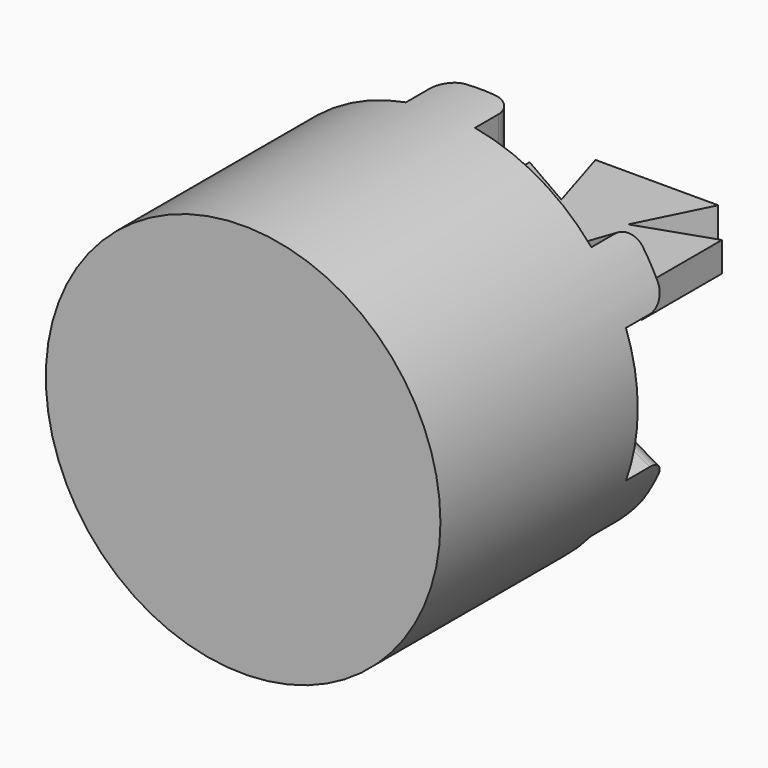
from build123d import *

# Parameters (mm, degrees)
F0_R     = 20
F1_DEPTH = 30
F2_R     = 15
F3_DEPTH = 10
F5_DEPTH = 5
F6_R     = 2
F8_DEPTH = 3


# Not quite as in the source:
# - a feature names something its author has since deleted; it is built from what else it names


with BuildPart() as f1:
    # F0 (on Front) → F1 (new body)
    with BuildSketch(Plane.XZ):
        Circle(F0_R)
    extrude(amount=-F1_DEPTH)

    # F2 (on face) → F3 (cut)
    with BuildSketch(Plane(origin=(0, 30, 0), x_dir=(-1, 0, 0), z_dir=(0, 1, 0))):
        Circle(F2_R)
    extrude(amount=-F3_DEPTH, mode=Mode.SUBTRACT)

    # F4 (on face) → F5 (cut)
    with BuildSketch(Plane(origin=(0, 30, 0), x_dir=(-1, 0, 0), z_dir=(0, 1, 0))):
        with BuildLine():
            Line((-3.5, -19.6913686675), (-3.5, -14.5859521458))
            ThreePointArc((-3.5, -14.5859521458), (-7.5, -12.9903810568), (-10.8818050967, -10.3240649862))
            Line((-10.8818050967, -10.3240649862), (-15.3032255014, -12.876773247))
            ThreePointArc((-15.3032255014, -12.876773247), (-10, -17.3205080757), (-3.5, -19.6913686675))
        make_face()
        with BuildLine():
            Line((-18.8032255014, -6.8145954205), (-14.3818050967, -4.2618871597))
            ThreePointArc((-14.3818050967, -4.2618871597), (-15, 0), (-14.3818050967, 4.2618871597))
            Line((-14.3818050967, 4.2618871597), (-18.8032255014, 6.8145954205))
            ThreePointArc((-18.8032255014, 6.8145954205), (-20, 0), (-18.8032255014, -6.8145954205))
        make_face()
        with BuildLine():
            Line((-15.3032255014, 12.876773247), (-10.8818050967, 10.3240649862))
            ThreePointArc((-10.8818050967, 10.3240649862), (-7.5, 12.9903810568), (-3.5, 14.5859521458))
            Line((-3.5, 14.5859521458), (-3.5, 19.6913686675))
            ThreePointArc((-3.5, 19.6913686675), (-10, 17.3205080757), (-15.3032255014, 12.876773247))
        make_face()
        with BuildLine():
            ThreePointArc((3.5, 14.5859521458), (7.5, 12.9903810568), (10.8818050967, 10.3240649862))
            Line((10.8818050967, 10.3240649862), (15.3032255014, 12.876773247))
            ThreePointArc((15.3032255014, 12.876773247), (10, 17.3205080757), (3.5, 19.6913686675))
            Line((3.5, 19.6913686675), (3.5, 14.5859521458))
        make_face()
        with BuildLine():
            ThreePointArc((15, 0), (14.8446467868, -2.1532444764), (14.3818050967, -4.2618871597))
            Line((14.3818050967, -4.2618871597), (18.8032255014, -6.8145954205))
            ThreePointArc((18.8032255014, -6.8145954205), (19.6985343367, -3.4594428723), (20, 0))
            ThreePointArc((20, 0), (19.6985343367, 3.4594428723), (18.8032255014, 6.8145954205))
            Line((18.8032255014, 6.8145954205), (14.3818050967, 4.2618871597))
            ThreePointArc((14.3818050967, 4.2618871597), (14.8446467868, 2.1532444764), (15, 0))
        make_face()
        with BuildLine():
            ThreePointArc((10.8818050967, -10.3240649862), (7.5, -12.9903810568), (3.5, -14.5859521458))
            Line((3.5, -14.5859521458), (3.5, -19.6913686675))
            ThreePointArc((3.5, -19.6913686675), (10, -17.3205080757), (15.3032255014, -12.876773247))
            Line((15.3032255014, -12.876773247), (10.8818050967, -10.3240649862))
        make_face()
    extrude(amount=-F5_DEPTH, mode=Mode.SUBTRACT)

    # F6
    f6_edges = [f1.edges().sort_by_distance(p)[0] for p in [
        (-3.5, 30, -17.13866),
        (3.5, 30, -17.13866),
        (13.092515, 30, -11.600419),
        (16.592515, 30, -5.538241),
        (16.592515, 30, 5.538241),
        (3.5, 30, 17.13866),
        (-3.5, 30, 17.13866),
        (-13.092515, 30, 11.600419),
        (-16.592515, 30, 5.538241),
        (-16.592515, 30, -5.538241),
        (-13.092515, 30, -11.600419),
        (13.092515, 30, 11.600419),
    ]]
    fillet(f6_edges, radius=F6_R)


with BuildPart() as f8:
    # F7 (on Top) → F8 (new body)
    with BuildSketch(Plane.XY):
        Polygon((-3.5101084504, 40.1726104319), (-3.5101084504, 30.1293712109), (3.2285826746, 30.1941670477), (3.2285826746, 39.9782285094), (10.744814761, 37.0624475181), (10.744814761, 47.2352765501), (3.2933775801, 44.7082668543), (6.7923129536, 51.7061389983), (-5.6483466178, 51.7061389983), (-3.5101084504, 44.7082668543), (-9.4712572172, 48.1424108148), (-9.4712572172, 37.0624475181), align=None)
    extrude(amount=F8_DEPTH)


solid = Compound([f1.part, f8.part])
